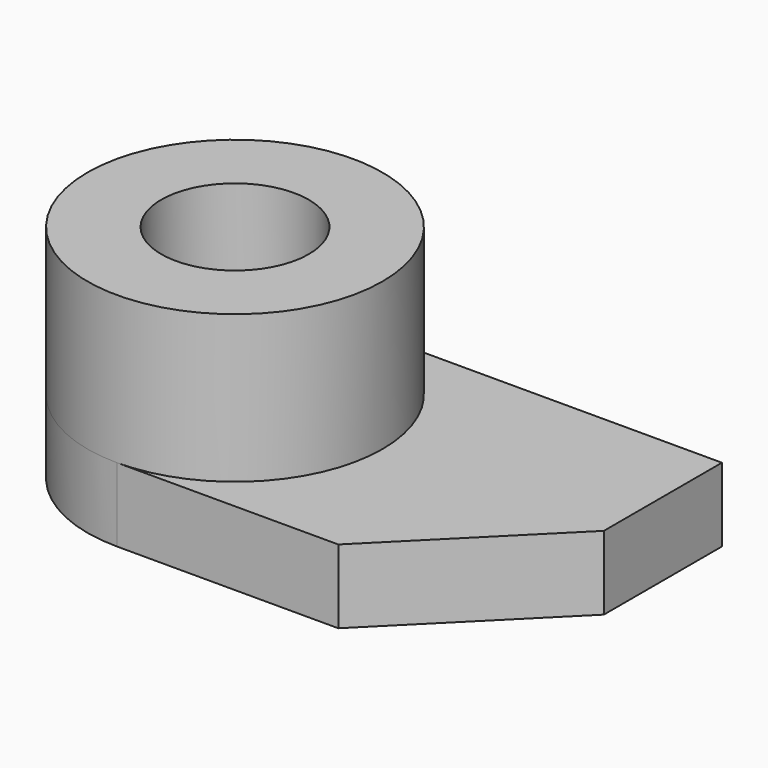
from build123d import *

# Parameters (mm, degrees)
F0_R     = 12.7
F0_R_2   = 6.35
F1_DEPTH = 12.7
F2_R     = 6.35
F3_DEPTH = 6.35


with BuildPart() as f1:
    # F0 (on Top) → F1 (new body)
    with BuildSketch(Plane.XY):
        Circle(F0_R)
        Circle(F0_R_2, mode=Mode.SUBTRACT)
    extrude(amount=-F1_DEPTH)

    # F2 (on face) → F3 (join)
    with BuildSketch(Plane(origin=(0, 0, -12.7), x_dir=(1, 0, 0), z_dir=(0, 0, -1))):
        with BuildLine():
            Line((19.05, 12.7), (0, 12.7))
            ThreePointArc((0, 12.7), (8.9802561211, 8.9802561211), (12.7, 0))
            ThreePointArc((12.7, 0), (8.9802561211, -8.9802561211), (0, -12.7))
            Line((0, -12.7), (31.75, -12.7))
            Line((31.75, -12.7), (31.75, 0))
            Line((31.75, 0), (19.05, 12.7))
        make_face()
        with BuildLine():
            ThreePointArc((12.7, 0), (8.9802561211, 8.9802561211), (0, 12.7))
            ThreePointArc((0, 12.7), (-12.7, 0), (0, -12.7))
            ThreePointArc((0, -12.7), (8.9802561211, -8.9802561211), (12.7, 0))
        make_face()
        Circle(F2_R, mode=Mode.SUBTRACT)
    extrude(amount=F3_DEPTH)


solid = f1.part
